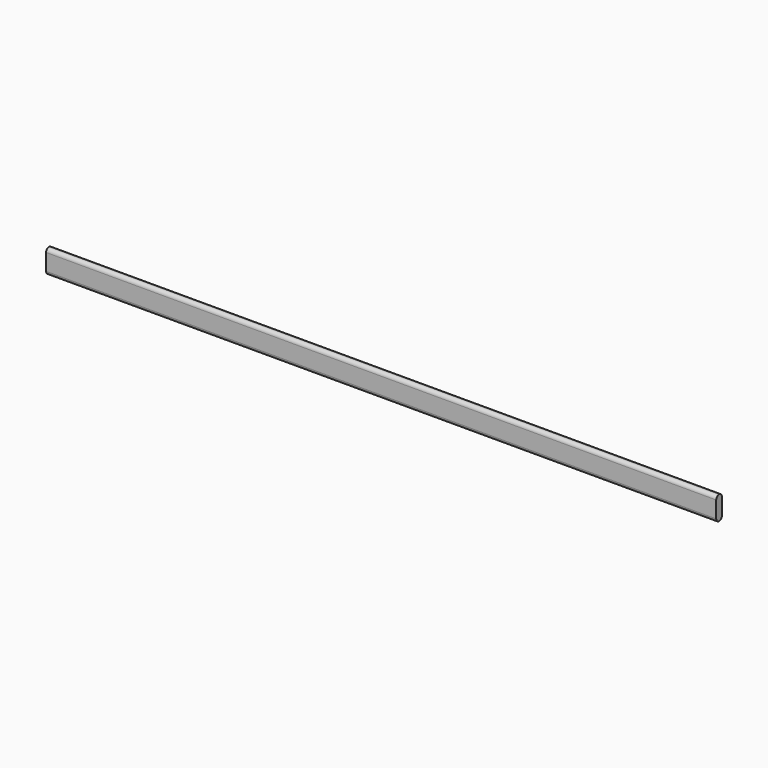
from build123d import *

# Parameters (mm, degrees)
F0_W     = 1797.05
F0_H     = 63.5
F1_DEPTH = 19.05
F2_R     = 9.52499


# Not quite as in the source:
# - a fillet or chamfer is up to 0.001 mm smaller than in the source, because OpenCascade refuses the exact size


with BuildPart() as f1:
    # F0 (on Front) → F1 (new body)
    with BuildSketch(Plane.XZ):
        with Locations((898.525, 31.75)):
            Rectangle(F0_W, F0_H)
    extrude(amount=F1_DEPTH)

    # F2 (radius 9.525 in the source; OpenCascade refuses exactly that, so slightly less here)
    f2_edges = [f1.edges().sort_by_distance(p)[0] for p in [
        (898.525, -19.05, 63.5),
        (898.525, 0, 63.5),
        (898.525, -19.05, 0),
        (898.525, 0, 0),
    ]]
    fillet(f2_edges, radius=F2_R)


solid = f1.part
